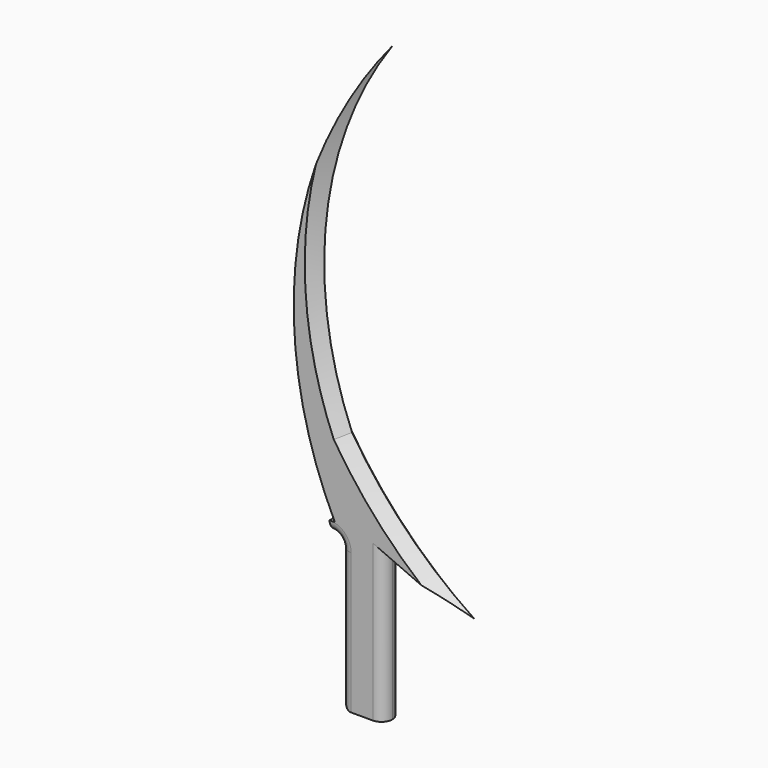
from build123d import *

# Parameters (mm, degrees)
F1_DEPTH     = 25.4
F2_T1_DEPTH  = 25.4
F2_T3_DEPTH  = 196.85
F2_T5_DEPTH  = 88.9
F2_T10_DEPTH = 241.3
F2_T15_DEPTH = 241.3
F2_T18_ANGLE = 233.2969892374
F2_T20_ANGLE = 233.2969892374
F3_C1_SIZE   = 12.7
F3_C2_SIZE   = 12.7
F3_C3_SIZE   = 12.6999
F3_C4_SIZE   = 12.6999


# Not quite as in the source:
# - a fillet or chamfer that OpenCascade refuses, or shapes differently, is made with other operations: its cross-section is extruded or revolved along the edge and cut away or added
# - a fillet or chamfer is up to 0.001 mm smaller than in the source, because OpenCascade refuses the exact size


with BuildPart() as f1:
    # F0 (on Front) → F1 (new body)
    with BuildSketch(Plane.XZ):
        Polygon((-25.4, -107.4178270914), (0, -107.4178270914), (25.4, -107.4178270914), (25.4, 70.3821729086), (-25.4, 70.3821729086), align=None)
        with BuildLine():
            ThreePointArc((-31.8772674395, 83.0821729086), (-28.6865783939, 76.7077201152), (-25.4, 70.3821729086))
            Line((-25.4, 70.3821729086), (25.4, 70.3821729086))
            Line((25.4, 70.3821729086), (46.7168006713, 61.0254222331))
            ThreePointArc((46.7168006713, 61.0254222331), (8.0726901659, 114.8632107301), (-21.8660467054, 173.9863600165))
            ThreePointArc((-21.8660467054, 173.9863600165), (-51.7756284743, 387.4903570682), (25.4, 588.7922751123))
            ThreePointArc((25.4, 588.7922751123), (-77.2246025315, 344.3169540256), (-31.8772674395, 83.0821729086))
        make_face()
        with BuildLine():
            Line((-38.1, 70.3821729086), (-25.4, 70.3821729086))
            ThreePointArc((-25.4, 70.3821729086), (-28.6865783939, 76.7077201152), (-31.8772674395, 83.0821729086))
            Line((-31.8772674395, 83.0821729086), (-38.1, 83.0821729086))
            Line((-38.1, 83.0821729086), (-38.1, 70.3821729086))
        make_face()
        with BuildLine():
            ThreePointArc((-21.8660467054, 173.9863600165), (8.0726901659, 114.8632107301), (46.7168006713, 61.0254222331))
            Line((46.7168006713, 61.0254222331), (121.4661896229, 28.2150860876))
            ThreePointArc((121.4661896229, 28.2150860876), (42.125694257, 93.5547531424), (-21.8660467054, 173.9863600165))
        make_face()
    extrude(amount=F1_DEPTH)

    # F2: fillet of radius 12.7 on 6 edges, made by hand

    # F2_s2 → F2_t1 (join)
    with BuildSketch(Plane.XZ):
        with BuildLine():
            ThreePointArc((-25.4, 57.6821729086), (-29.1197438789, 66.6624290297), (-38.1, 70.3821729086))
            Line((-38.1, 70.3821729086), (-25.4, 70.3821729086))
            Line((-25.4, 70.3821729086), (-25.4, 57.6821729086))
        make_face()
    extrude(amount=F2_T1_DEPTH)

    # F2_s4 → F2_t3 (cut)
    with BuildSketch(Plane.XY.offset(-139.1678270914)):
        with BuildLine():
            ThreePointArc((-25.4, -12.7), (-21.6802561211, -3.7197438789), (-12.7, 0))
            Line((-12.7, 0), (-25.4, 0))
            Line((-25.4, 0), (-25.4, -12.7))
        make_face()
        with BuildLine():
            ThreePointArc((-25.4, -12.7), (-21.6802561211, -21.6802561211), (-12.7, -25.4))
            Line((-12.7, -25.4), (-25.4, -25.4))
            Line((-25.4, -25.4), (-25.4, -12.7))
        make_face()
    extrude(amount=F2_T3_DEPTH, mode=Mode.SUBTRACT)

    # F2_s6 → F2_t5 (cut)
    with BuildSketch(Plane.XZ.offset(-31.75)):
        with BuildLine():
            ThreePointArc((-25.4, -94.7178270914), (-21.6802561211, -103.6980832124), (-12.7, -107.4178270914))
            Line((-12.7, -107.4178270914), (-25.4, -107.4178270914))
            Line((-25.4, -107.4178270914), (-25.4, -94.7178270914))
        make_face()
    extrude(amount=F2_T5_DEPTH, mode=Mode.SUBTRACT)


with BuildPart() as f2_tool8:
    # F2_s9 → F2_t10 (new body)
    with BuildSketch(Plane.XY.offset(-139.1678270914)):
        with BuildLine():
            ThreePointArc((12.7, 0), (21.6802561211, -3.7197438789), (25.4, -12.7))
            Line((25.4, -12.7), (25.4, 0))
            Line((25.4, 0), (12.7, 0))
        make_face()
    extrude(amount=F2_T10_DEPTH)

    split(bisect_by=Plane(origin=(30.005981648, 0, 68.3604332226), x_dir=(0, 1, 0), z_dir=(-0.4019236244, 0, -0.9156731951)), keep=Keep.TOP)


with BuildPart() as f1_1:
    add(f1.part)

    # F2_t7: cut F2_tool8
    add(f2_tool8.part, mode=Mode.SUBTRACT)


with BuildPart() as f2_tool13:
    # F2_s14 → F2_t15 (new body)
    with BuildSketch(Plane.XY.offset(-139.1678270914)):
        with BuildLine():
            ThreePointArc((12.7, -25.4), (21.6802561211, -21.6802561211), (25.4, -12.7))
            Line((25.4, -12.7), (25.4, -25.4))
            Line((25.4, -25.4), (12.7, -25.4))
        make_face()
    extrude(amount=F2_T15_DEPTH)

    split(bisect_by=Plane(origin=(30.005981648, 0, 68.3604332226), x_dir=(0, 1, 0), z_dir=(-0.4019236244, 0, -0.9156731951)), keep=Keep.TOP)


with BuildPart() as f1_2:
    add(f1_1.part)

    # F2_t12: cut F2_tool13
    add(f2_tool13.part, mode=Mode.SUBTRACT)

    # F2_s17 → F2_t18 (revolve, cut)
    with BuildSketch(Plane.XY.offset(57.6821729086)):
        with BuildLine():
            ThreePointArc((-12.7, -25.4), (-21.6802561211, -21.6802561211), (-25.4, -12.7))
            Line((-25.4, -12.7), (-25.4, -25.4))
            Line((-25.4, -25.4), (-12.7, -25.4))
        make_face()
    revolve(axis=Axis((-38.1, -25.4, 57.6821729086), (0, -1, 0)), revolution_arc=F2_T18_ANGLE, mode=Mode.SUBTRACT)

    # F2_s19 → F2_t20 (revolve, cut)
    with BuildSketch(Plane.XY.offset(57.6821729086)):
        with BuildLine():
            ThreePointArc((-12.7, 0), (-21.6802561211, -3.7197438789), (-25.4, -12.7))
            Line((-25.4, -12.7), (-25.4, 0))
            Line((-25.4, 0), (-12.7, 0))
        make_face()
    revolve(axis=Axis((-38.1, 0, 57.6821729086), (0, -1, 0)), revolution_arc=F2_T20_ANGLE, mode=Mode.SUBTRACT)

    # F3: chamfer of 12.7 on 4 edges, made by hand

    # F3_c1
    f3_c1_edges = [f1_2.edges().sort_by_distance(p)[0] for p in [
        (-51.7756284743, 0, 387.4903570682),
    ]]
    chamfer(f3_c1_edges, length=F3_C1_SIZE)

    # F3_c2
    f3_c2_edges = [f1_2.edges().sort_by_distance(p)[0] for p in [
        (42.125694257, 0, 93.5547531424),
    ]]
    chamfer(f3_c2_edges, length=F3_C2_SIZE)

    # F3_c3 (size 12.7 in the source; OpenCascade refuses exactly that, so slightly less here)
    f3_c3_edges = [f1_2.edges().sort_by_distance(p)[0] for p in [
        (-51.7756284743, -25.4, 387.4903570682),
    ]]
    chamfer(f3_c3_edges, length=F3_C3_SIZE)

    # F3_c4 (size 12.7 in the source; OpenCascade refuses exactly that, so slightly less here)
    f3_c4_edges = [f1_2.edges().sort_by_distance(p)[0] for p in [
        (42.125694257, -25.4, 93.5547531424),
    ]]
    chamfer(f3_c4_edges, length=F3_C4_SIZE)


solid = f1_2.part
